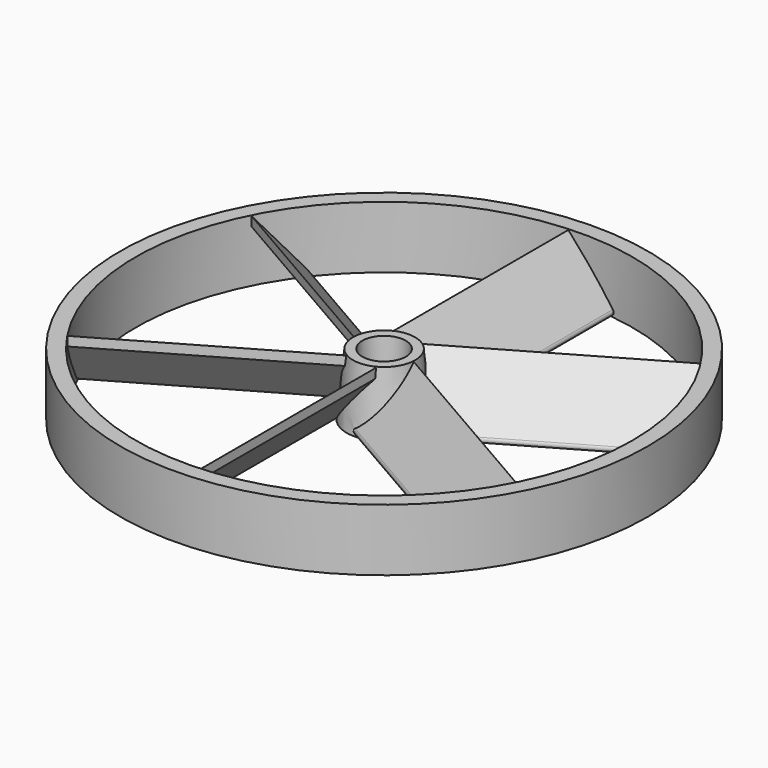
from build123d import *

# Parameters (mm, degrees)
F0_R         = 7.62
F2_R         = 6.35
F6_R         = 53.975
F6_R_2       = 50.8
F7_DEPTH     = 12.7
F9_DEPTH     = 52.95041
F10_T1_DEPTH = 51.2091039216
F10_T3_DEPTH = 49.5691829778
F12_COUNT    = 6
F4_R         = 4.064
F5_R         = 4.445


# Not quite as in the source:
# - a fillet or chamfer that OpenCascade refuses, or shapes differently, is made with other operations: its cross-section is extruded or revolved along the edge and cut away or added


with BuildPart() as f3:
    # F0 (on Top) → F3 section 0
    with BuildSketch(Plane.XY):
        Circle(F0_R)
    # F2 (on offset) → F3 section 1
    with BuildSketch(Plane.XY.offset(12.7)):
        Circle(F2_R)
    loft()



with BuildPart() as f7:
    # F6 (on Top) → F7 (new body)
    with BuildSketch(Plane.XY):
        Circle(F6_R)
        Circle(F6_R_2, mode=Mode.SUBTRACT)
    extrude(amount=F7_DEPTH)


with BuildPart() as f3_1:
    add(f3.part)

    add(f7.part)  # F9 merges F7
    # F8 (on Front) → F9 (join)
    with BuildSketch(Plane.XZ):
        Polygon((-6.951478799, 0.7896896311), (-6.0103633441, 0), (2.8918089811, 10.6091958504), (2.8918089811, 12.5204632059), align=None)
    extrude(amount=F9_DEPTH)

    # F10: fillet of radius 0.762 on 2 edges, made by hand

    # F10_s2 → F10_t1 (cut)
    with BuildSketch(Plane.XZ.offset(1.0180278149)):
        with BuildLine():
            ThreePointArc((-6.3677529333, 0.2998854725), (-6.6370491347, 0.8171986622), (-6.4616746404, 1.3734154967))
            Line((-6.4616746404, 1.3734154967), (-6.4733491577, 1.3832115799))
            Line((-6.4733491577, 1.3832115799), (-6.9729493995, 0.7878111969))
            Line((-6.9729493995, 0.7878111969), (-6.3775490165, 0.2882109552))
            Line((-6.3775490165, 0.2882109552), (-6.3677529333, 0.2998854725))
        make_face()
    extrude(amount=F10_T1_DEPTH, mode=Mode.SUBTRACT)

    # F10_s4 → F10_t3 (cut)
    with BuildSketch(Plane.XZ.offset(2.7790081631)):
        with BuildLine():
            ThreePointArc((-6.5940892098, 0.4898041586), (-6.0378723752, 0.3144296643), (-5.5205591855, 0.5837258657))
            Line((-5.5205591855, 0.5837258657), (-5.5088846682, 0.5739297825))
            Line((-5.5088846682, 0.5739297825), (-6.00848491, -0.0214706005))
            Line((-6.00848491, -0.0214706005), (-6.6038852929, 0.4781296413))
            Line((-6.6038852929, 0.4781296413), (-6.5940892098, 0.4898041586))
        make_face()
    extrude(amount=F10_T3_DEPTH, mode=Mode.SUBTRACT)

    # F12: F3 ×6 about axis
    f12_axis = Axis((0, 0, 18.5918267816), (0, 0, 1))


with BuildPart() as f3_2:
    add(f3_1.part)
    for i in range(1, F12_COUNT):
        add(f3_1.part.rotate(f12_axis, i * 360 / F12_COUNT))

    # F4 (on Top) → F13 section 0
    with BuildSketch(Plane.XY):
        Circle(F4_R)
    # F5 (on offset) → F13 section 1
    with BuildSketch(Plane.XY.offset(12.7)):
        Circle(F5_R)
    loft(mode=Mode.SUBTRACT)


solid = f3_2.part
